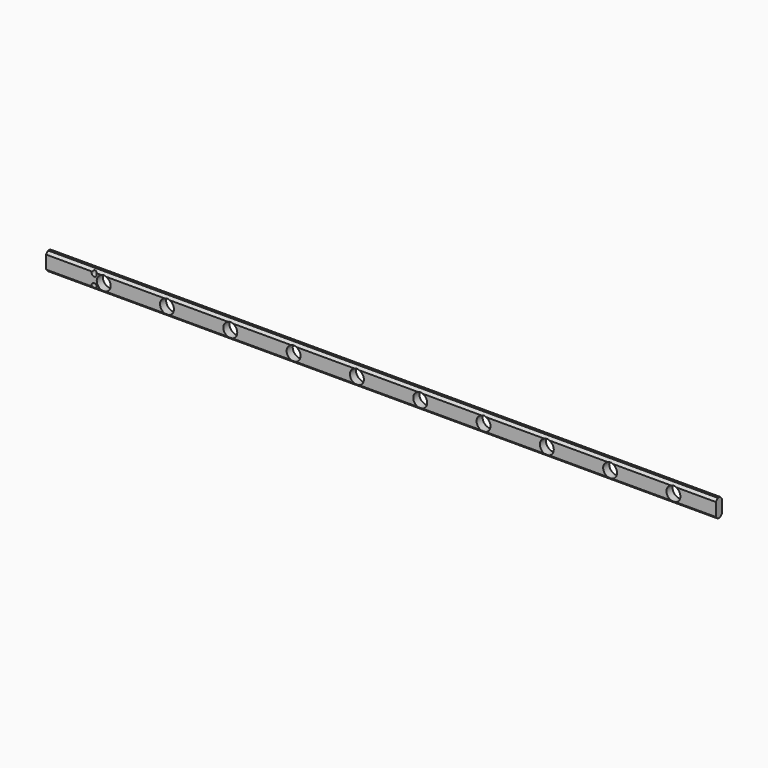
from build123d import *

# Parameters (mm, degrees)
F0_W        = 264.5
F0_H        = 7.2
F0_R        = 1
F0_R_2      = 2.75
F1_DEPTH    = 3
F2_T1_DEPTH = 269.6433659759


# Not quite as in the source:
# - a fillet or chamfer that OpenCascade refuses, or shapes differently, is made with other operations: its cross-section is extruded or revolved along the edge and cut away or added


with BuildPart() as f1:
    # F0 (on Front) → F1 (new body)
    with BuildSketch(Plane.XZ):
        Rectangle(F0_W, F0_H)
        with Locations((-113.25, -2.1)):
            Circle(F0_R, mode=Mode.SUBTRACT)
        with Locations((-109.5, 0)):
            Circle(F0_R_2, mode=Mode.SUBTRACT)
        with Locations((-84.5, 0)):
            Circle(F0_R_2, mode=Mode.SUBTRACT)
        with Locations((-59.5, 0)):
            Circle(F0_R_2, mode=Mode.SUBTRACT)
        with Locations((-34.5, 0)):
            Circle(F0_R_2, mode=Mode.SUBTRACT)
        with Locations((-9.5, 0)):
            Circle(F0_R_2, mode=Mode.SUBTRACT)
        with Locations((-113.25, 2.1)):
            Circle(F0_R, mode=Mode.SUBTRACT)
        with Locations((15.5, 0)):
            Circle(F0_R_2, mode=Mode.SUBTRACT)
        with Locations((40.5, 0)):
            Circle(F0_R_2, mode=Mode.SUBTRACT)
        with Locations((65.5, 0)):
            Circle(F0_R_2, mode=Mode.SUBTRACT)
        with Locations((90.5, 0)):
            Circle(F0_R_2, mode=Mode.SUBTRACT)
        with Locations((115.5, 0)):
            Circle(F0_R_2, mode=Mode.SUBTRACT)
    extrude(amount=F1_DEPTH)

    # F2: chamfer of 1 on 4 edges, made by hand

    # F2_s2 → F2_t1 (cut)
    with BuildSketch(Plane.YZ.offset(-134.821682988)):
        Polygon((-2, -3.6), (-3, -2.6), (-3, -3.6), align=None)
        Polygon((-1, -3.6), (0, -2.6), (0, -3.6), align=None)
        Polygon((-1, 3.6), (0, 2.6), (0, 3.6), align=None)
        Polygon((-2, 3.6), (-3, 2.6), (-3, 3.6), align=None)
    extrude(amount=F2_T1_DEPTH, mode=Mode.SUBTRACT)


solid = f1.part
